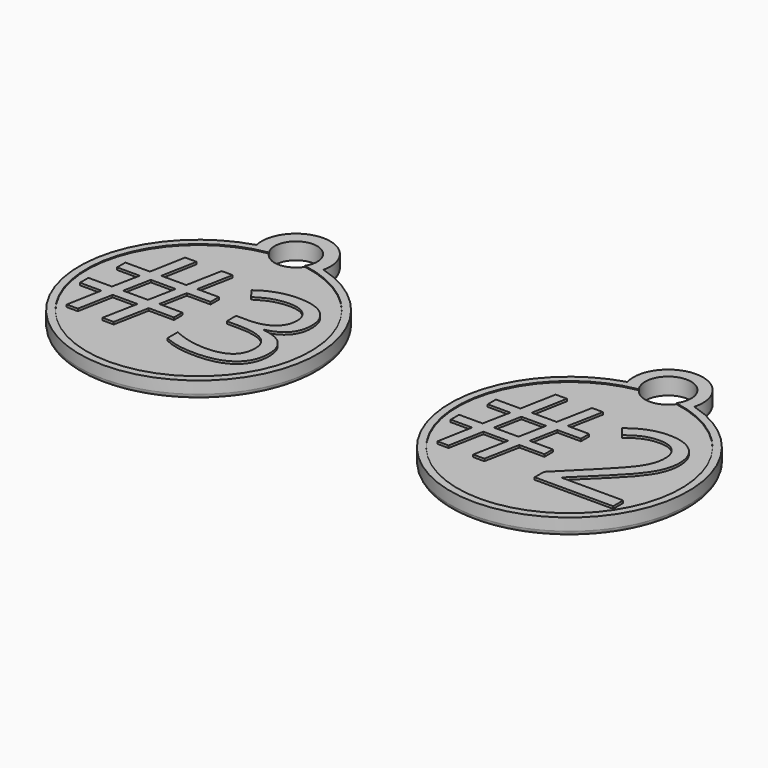
from build123d import *

# Parameters (mm, degrees)
F0_R           = 4.589425573
F1_DEPTH       = 3.6
F0_R_2         = 4.9476301443
F2_R           = 1
F2_2_R         = 1
F4_R           = 24.1315176083
F5_DEPTH       = 0.2
F6_TEXT_SIZE   = 36.1999254712
F6_TEXT_SIZE_2 = 36.0903353943
F7_DEPTH       = 0.5


# Not quite as in the source:
# - Text() gives the source's letters only with a copy of the font that has no kerning and outlines rounded to 1/6400 em; it was checked with that copy


with BuildPart() as f1:
    # F0 (on Top) → F1 (new body)
    with BuildSketch(Plane.XY):
        with BuildLine():
            ThreePointArc((-32.7659994364, 37.2110009193), (-40.0050003082, 46.2205437645), (-47.2440011799, 37.2110009193))
            ThreePointArc((-47.2440011799, 37.2110009193), (-40.0050003082, -13.1516965924), (-32.7659994364, 37.2110009193))
        make_face()
        with Locations((-40.0050003082, 38.8075707537)):
            Circle(F0_R, mode=Mode.SUBTRACT)
    extrude(amount=F1_DEPTH)

    # F2
    f2_edges = [f1.edges().sort_by_distance(p)[0] for p in [
        (-40.005, -13.151697, 0),
        (-40.005, 46.220544, 0),
    ]]
    fillet(f2_edges, radius=F2_R)


with BuildPart() as f1b:
    # F0 (on Top) → F1, piece 2 (new body)
    with BuildSketch(Plane.XY):
        with BuildLine():
            ThreePointArc((32.7659994364, 37.2110009193), (40.0050003082, -13.1516965924), (47.2440011799, 37.2110009193))
            ThreePointArc((47.2440011799, 37.2110009193), (40.0050003082, 46.6965480463), (32.7659994364, 37.2110009193))
        make_face()
        with Locations((40.0050003082, 39.1915124372)):
            Circle(F0_R_2, mode=Mode.SUBTRACT)
    extrude(amount=F1_DEPTH)

    # F2#2
    f2_2_edges = [f1b.edges().sort_by_distance(p)[0] for p in [
        (40.005, -13.151697, 0),
        (40.005, 46.696548, 0),
    ]]
    fillet(f2_2_edges, radius=F2_2_R)


with BuildPart() as f5_tool:
    # F4 (on face) → F5 (new body)
    with BuildSketch(Plane.XY.offset(3.6)):
        with Locations((-40.0050003082, 12.5499095783)):
            Circle(F4_R)
        with Locations((40.0050003082, 12.5499095783)):
            Circle(F4_R)
    extrude(amount=-F5_DEPTH)


with BuildPart() as f1_1:
    add(f1.part)

    # F5: cut by f5_tool
    add(f5_tool.part, mode=Mode.SUBTRACT)


with BuildPart() as f1b_1:
    add(f1b.part)

    # F5: cut by f5_tool
    add(f5_tool.part, mode=Mode.SUBTRACT)


with BuildPart() as f7:
    # F6 (on face) → F7 (new body)
    with BuildSketch(Plane.XY.offset(3.6)):
        with Locations((-62.157657825, -0.4820635913)):
            Text('#3', F6_TEXT_SIZE, font='Open Sans', text_align=(TextAlign.LEFT, TextAlign.BOTTOM))
        with Locations((17.8291809429, -0.4426111636)):
            Text('#2', F6_TEXT_SIZE_2, font='Open Sans', text_align=(TextAlign.LEFT, TextAlign.BOTTOM))
    extrude(amount=F7_DEPTH)


solid = Compound([f1_1.part, f1b_1.part, f7.part])
